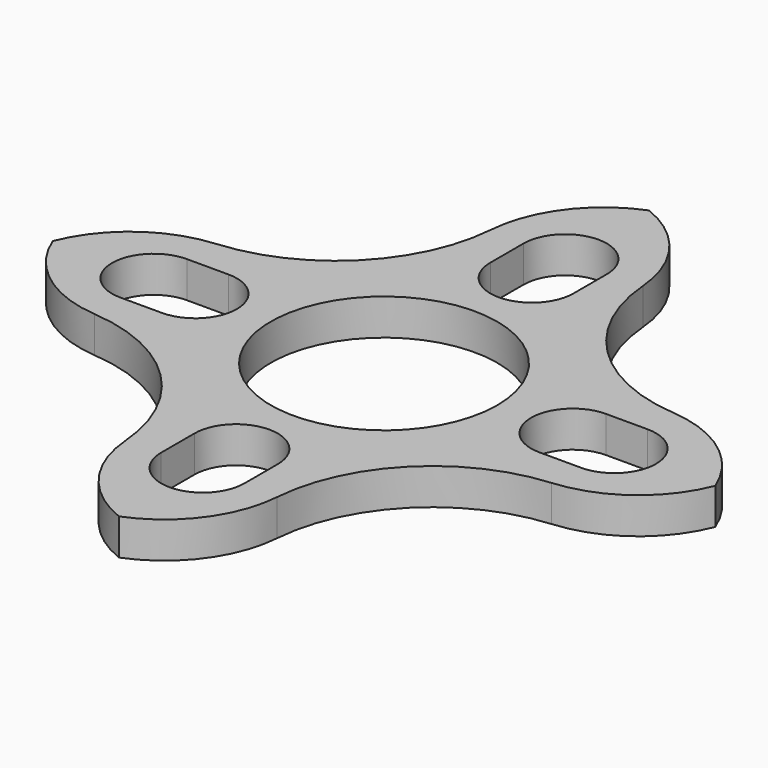
from build123d import *

# Parameters (mm, degrees)
F0_R        = 1.75
F1_DEPTH    = 1.524
F2_R        = 6.985
F3_T1_DEPTH = 26.7357127365
F4_R        = 4.7625
F5_DEPTH    = 25.4


# Not quite as in the source:
# - a fillet or chamfer that OpenCascade refuses, or shapes differently, is made with other operations: its cross-section is extruded or revolved along the edge and cut away or added


with BuildPart() as f1:
    # F0 (on Top) → F1 (new body)
    with BuildSketch(Plane.XY):
        Polygon((3.175, 3.175), (3.175, 14.2875), (-3.175, 14.2875), (-3.175, 3.175), (-14.2875, 3.175), (-14.2875, -3.175), (-3.175, -3.175), (-3.175, -14.2875), (3.175, -14.2875), (3.175, -3.175), (14.2875, -3.175), (14.2875, 3.175), align=None)
        with BuildLine():
            ThreePointArc((1.75, -9.525), (-1.2374368671, -10.7624368671), (0, -7.775))
            ThreePointArc((0, -7.775), (1.2374368671, -8.2875631329), (1.75, -9.525))
        make_face(mode=Mode.SUBTRACT)
        with Locations((-7.9375, 0)):
            Circle(F0_R, mode=Mode.SUBTRACT)
        with BuildLine():
            ThreePointArc((9.6875, 0), (7.9375, -1.75), (6.1875, 0))
            ThreePointArc((6.1875, 0), (7.9375, 1.75), (9.6875, 0))
        make_face(mode=Mode.SUBTRACT)
        with BuildLine():
            ThreePointArc((0, 7.775), (-1.2374368671, 10.7624368671), (1.75, 9.525))
            ThreePointArc((1.75, 9.525), (1.2374368671, 8.2875631329), (0, 7.775))
        make_face(mode=Mode.SUBTRACT)
    extrude(amount=F1_DEPTH)

    # F2
    f2_edges = [f1.edges().sort_by_distance(p)[0] for p in [
        (3.175, -3.175, 0.762),
        (-3.175, 3.175, 0.762),
        (3.175, 3.175, 0.762),
        (-3.175, -3.175, 0.762),
    ]]
    fillet(f2_edges, radius=F2_R)

    # F3: fillet of radius 5.08 on 8 edges, made by hand

    # F3_s2 → F3_t1 (cut)
    with BuildSketch(Plane.XY.offset(-12.6058563682)):
        with BuildLine():
            ThreePointArc((3.1968016831, 9.6085526316), (1.5800515868, 12.9387027128), (-1.8673425473, 14.2875))
            Line((-1.8673425473, 14.2875), (-1.8673425473, 14.7955))
            Line((-1.8673425473, 14.7955), (3.175, 14.7955))
            Line((3.175, 14.7955), (3.683, 14.2875))
            ThreePointArc((3.683, 14.2875), (3.683, 10.16), (3.7032161062, 9.6486578947))
            Line((3.7032161062, 9.6486578947), (3.1968016831, 9.6085526316))
        make_face()
        with BuildLine():
            ThreePointArc((1.8673425473, 14.2875), (-1.5800515868, 12.9387027128), (-3.1968016831, 9.6085526316))
            Line((-3.1968016831, 9.6085526316), (-3.7032161062, 9.6486578947))
            ThreePointArc((-3.7032161062, 9.6486578947), (-3.683, 10.16), (-3.683, 14.2875))
            Line((-3.683, 14.2875), (-3.175, 14.7955))
            Line((-3.175, 14.7955), (1.8673425473, 14.7955))
            Line((1.8673425473, 14.7955), (1.8673425473, 14.2875))
        make_face()
        with BuildLine():
            ThreePointArc((-14.2875, 1.8673425473), (-12.9387027128, -1.5800515868), (-9.6085526316, -3.1968016831))
            Line((-9.6085526316, -3.1968016831), (-9.6486578947, -3.7032161062))
            ThreePointArc((-9.6486578947, -3.7032161062), (-10.16, -3.683), (-14.2875, -3.683))
            Line((-14.2875, -3.683), (-14.7955, -3.175))
            Line((-14.7955, -3.175), (-14.7955, 1.8673425473))
            Line((-14.7955, 1.8673425473), (-14.2875, 1.8673425473))
        make_face()
        with BuildLine():
            ThreePointArc((-9.6085526316, 3.1968016831), (-12.9387027128, 1.5800515868), (-14.2875, -1.8673425473))
            Line((-14.2875, -1.8673425473), (-14.7955, -1.8673425473))
            Line((-14.7955, -1.8673425473), (-14.7955, 3.175))
            Line((-14.7955, 3.175), (-14.2875, 3.683))
            ThreePointArc((-14.2875, 3.683), (-10.16, 3.683), (-9.6486578947, 3.7032161062))
            Line((-9.6486578947, 3.7032161062), (-9.6085526316, 3.1968016831))
        make_face()
        with BuildLine():
            ThreePointArc((1.8673425473, -14.2875), (-1.5800515868, -12.9387027128), (-3.1968016831, -9.6085526316))
            Line((-3.1968016831, -9.6085526316), (-3.7032161062, -9.6486578947))
            ThreePointArc((-3.7032161062, -9.6486578947), (-3.683, -10.16), (-3.683, -14.2875))
            Line((-3.683, -14.2875), (-3.175, -14.7955))
            Line((-3.175, -14.7955), (1.8673425473, -14.7955))
            Line((1.8673425473, -14.7955), (1.8673425473, -14.2875))
        make_face()
        with BuildLine():
            ThreePointArc((3.1968016831, -9.6085526316), (1.5800515868, -12.9387027128), (-1.8673425473, -14.2875))
            Line((-1.8673425473, -14.2875), (-1.8673425473, -14.7955))
            Line((-1.8673425473, -14.7955), (3.175, -14.7955))
            Line((3.175, -14.7955), (3.683, -14.2875))
            ThreePointArc((3.683, -14.2875), (3.683, -10.16), (3.7032161062, -9.6486578947))
            Line((3.7032161062, -9.6486578947), (3.1968016831, -9.6085526316))
        make_face()
        with BuildLine():
            ThreePointArc((14.2875, 1.8673425473), (12.9387027128, -1.5800515868), (9.6085526316, -3.1968016831))
            Line((9.6085526316, -3.1968016831), (9.6486578947, -3.7032161062))
            ThreePointArc((9.6486578947, -3.7032161062), (10.16, -3.683), (14.2875, -3.683))
            Line((14.2875, -3.683), (14.7955, -3.175))
            Line((14.7955, -3.175), (14.7955, 1.8673425473))
            Line((14.7955, 1.8673425473), (14.2875, 1.8673425473))
        make_face()
        with BuildLine():
            ThreePointArc((9.6085526316, 3.1968016831), (12.9387027128, 1.5800515868), (14.2875, -1.8673425473))
            Line((14.2875, -1.8673425473), (14.7955, -1.8673425473))
            Line((14.7955, -1.8673425473), (14.7955, 3.175))
            Line((14.7955, 3.175), (14.2875, 3.683))
            ThreePointArc((14.2875, 3.683), (10.16, 3.683), (9.6486578947, 3.7032161062))
            Line((9.6486578947, 3.7032161062), (9.6085526316, 3.1968016831))
        make_face()
    extrude(amount=F3_T1_DEPTH, mode=Mode.SUBTRACT)

    # F4 (on face) → F5 (cut)
    with BuildSketch(Plane.XY.offset(1.524)):
        Circle(F4_R)
        with BuildLine():
            ThreePointArc((1.75, 9.525), (0, 11.275), (-1.75, 9.525))
            Line((-1.75, 9.525), (-1.75, 7.775))
            ThreePointArc((-1.75, 7.775), (0, 6.025), (1.75, 7.775))
            Line((1.75, 7.775), (1.75, 9.525))
        make_face()
        with BuildLine():
            ThreePointArc((-1.75, -9.525), (0, -11.275), (1.75, -9.525))
            Line((1.75, -9.525), (1.75, -7.775))
            ThreePointArc((1.75, -7.775), (0, -6.025), (-1.75, -7.775))
            Line((-1.75, -7.775), (-1.75, -9.525))
        make_face()
        with BuildLine():
            ThreePointArc((7.9375, 1.75), (6.1875, 0), (7.9375, -1.75))
            Line((7.9375, -1.75), (9.6875, -1.75))
            ThreePointArc((9.6875, -1.75), (11.4375, 0), (9.6875, 1.75))
            Line((9.6875, 1.75), (7.9375, 1.75))
        make_face()
        with BuildLine():
            ThreePointArc((-7.9375, -1.75), (-6.1875, 0), (-7.9375, 1.75))
            Line((-7.9375, 1.75), (-9.6875, 1.75))
            ThreePointArc((-9.6875, 1.75), (-11.4375, 0), (-9.6875, -1.75))
            Line((-9.6875, -1.75), (-7.9375, -1.75))
        make_face()
    extrude(amount=-F5_DEPTH, mode=Mode.SUBTRACT)


solid = f1.part
